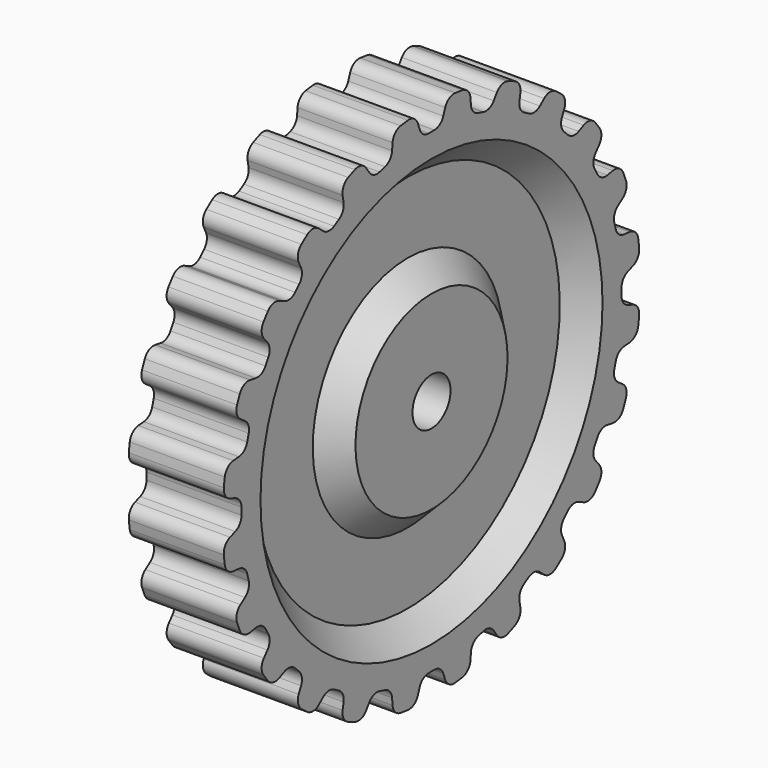
from build123d import *

# Parameters (mm, degrees)
F2_R            = 3.175
F3_DEPTH        = 12.701
F5_DEPTH        = 12.701
F5_COPIES_COUNT = 24
F6_R            = 1.5875


# Not quite as in the source:
# - a pattern or mirror of a feature is missing from the dataset's text; its kind, count and spacing are read off the source's solid


with BuildPart() as f1:
    # F0 (on Front) → F1 (revolve)
    with BuildSketch(Plane.XZ):
        Polygon((6.35, 34.925), (0, 34.925), (-6.35, 34.925), (-6.35, 28.575), (-3.175, 25.4), (-3.175, 15.875), (-6.35, 12.7), (-6.35, 0), (6.35, 0), (6.35, 12.7), (3.175, 15.875), (3.175, 25.4), (6.35, 28.575), align=None)
    revolve(axis=Axis((-0.6392432713, 0, 0), (1, 0, 0)))

    # F2 (on face) → F3 (cut, through all)
    with BuildSketch(Plane.YZ.offset(6.35)):
        Circle(F2_R)
    extrude(amount=-F3_DEPTH, mode=Mode.SUBTRACT)

    # F4 (on face) → F5 (cut, through all)
    with BuildSketch(Plane.YZ.offset(6.35)):
        with BuildLine():
            Line((1.5875, 31.75), (2.7049231948, 34.8200949957))
            ThreePointArc((2.7049231948, 34.8200949957), (0, 34.925), (-2.7049231948, 34.8200949957))
            Line((-2.7049231948, 34.8200949957), (-1.5875, 31.75))
            Line((-1.5875, 31.75), (0, 31.75))
            Line((0, 31.75), (1.5875, 31.75))
        make_face()
    f5 = extrude(amount=-F5_DEPTH, mode=Mode.SUBTRACT)

    # F5_copies: F5 ×24 about axis
    f5_copies_axis = Axis((0, 0, 0), (1, 0, 0))
    for i in range(1, F5_COPIES_COUNT):
        add(f5.rotate(f5_copies_axis, i * 360 / F5_COPIES_COUNT), mode=Mode.SUBTRACT)

    # F6
    f6_edges = [f1.edges().sort_by_distance(p)[0] for p in [
        (0, -1.5875, 31.75),
        (0, 1.5875, 31.75),
        (0, 2.704923, 34.820095),
        (0, -2.704923, 34.820095),
        (0, -6.399349, 34.333715),
        (0, -6.684097, 31.07902),
        (0, 6.399349, 34.333715),
        (0, 6.684097, 31.07902),
        (0, 9.750912, 30.25727),
        (0, 11.624859, 32.933543),
        (0, 15.067515, 31.507548),
        (0, 14.500185, 28.290057),
        (0, 17.249815, 26.702557),
        (0, 19.75258, 28.802625),
        (0, 22.708856, 26.534195),
        (0, 21.328108, 23.573172),
        (0, 23.573172, 21.328108),
        (0, 26.534195, 22.708856),
        (0, 28.802625, 19.75258),
        (0, 26.702557, 17.249815),
        (0, 28.290057, 14.500185),
        (0, 31.507548, 15.067515),
        (0, 32.933543, 11.624859),
        (0, 30.25727, 9.750912),
        (0, 31.07902, 6.684097),
        (0, 34.333715, 6.399349),
        (0, 34.820095, 2.704923),
        (0, 31.75, 1.5875),
        (0, 31.75, -1.5875),
        (0, 34.820095, -2.704923),
        (0, 34.333715, -6.399349),
        (0, 31.07902, -6.684097),
        (0, 30.25727, -9.750912),
        (0, 32.933543, -11.624859),
        (0, 31.507548, -15.067515),
        (0, 28.290057, -14.500185),
        (0, 26.702557, -17.249815),
        (0, 28.802625, -19.75258),
        (0, 26.534195, -22.708856),
        (0, 23.573172, -21.328108),
        (0, 21.328108, -23.573172),
        (0, 22.708856, -26.534195),
        (0, 19.75258, -28.802625),
        (0, 17.249815, -26.702557),
        (0, 14.500185, -28.290057),
        (0, 15.067515, -31.507548),
        (0, 11.624859, -32.933543),
        (0, 9.750912, -30.25727),
        (0, 6.684097, -31.07902),
        (0, 6.399349, -34.333715),
        (0, 2.704923, -34.820095),
        (0, 1.5875, -31.75),
        (0, -1.5875, -31.75),
        (0, -2.704923, -34.820095),
        (0, -6.399349, -34.333715),
        (0, -6.684097, -31.07902),
        (0, -9.750912, -30.25727),
        (0, -11.624859, -32.933543),
        (0, -15.067515, -31.507548),
        (0, -14.500185, -28.290057),
        (0, -17.249815, -26.702557),
        (0, -19.75258, -28.802625),
        (0, -22.708856, -26.534195),
        (0, -21.328108, -23.573172),
        (0, -23.573172, -21.328108),
        (0, -26.534195, -22.708856),
        (0, -28.802625, -19.75258),
        (0, -26.702557, -17.249815),
        (0, -28.290057, -14.500185),
        (0, -31.507548, -15.067515),
        (0, -32.933543, -11.624859),
        (0, -30.25727, -9.750912),
        (0, -31.07902, -6.684097),
        (0, -34.333715, -6.399349),
        (0, -34.820095, -2.704923),
        (0, -31.75, -1.5875),
        (0, -31.75, 1.5875),
        (0, -34.820095, 2.704923),
        (0, -34.333715, 6.399349),
        (0, -31.07902, 6.684097),
        (0, -30.25727, 9.750912),
        (0, -32.933543, 11.624859),
        (0, -31.507548, 15.067515),
        (0, -28.290057, 14.500185),
        (0, -26.702557, 17.249815),
        (0, -28.802625, 19.75258),
        (0, -26.534195, 22.708856),
        (0, -23.573172, 21.328108),
        (0, -21.328108, 23.573172),
        (0, -22.708856, 26.534195),
        (0, -19.75258, 28.802625),
        (0, -17.249815, 26.702557),
        (0, -14.500185, 28.290057),
        (0, -15.067515, 31.507548),
        (0, -11.624859, 32.933543),
        (0, -9.750912, 30.25727),
    ]]
    fillet(f6_edges, radius=F6_R)


solid = f1.part
